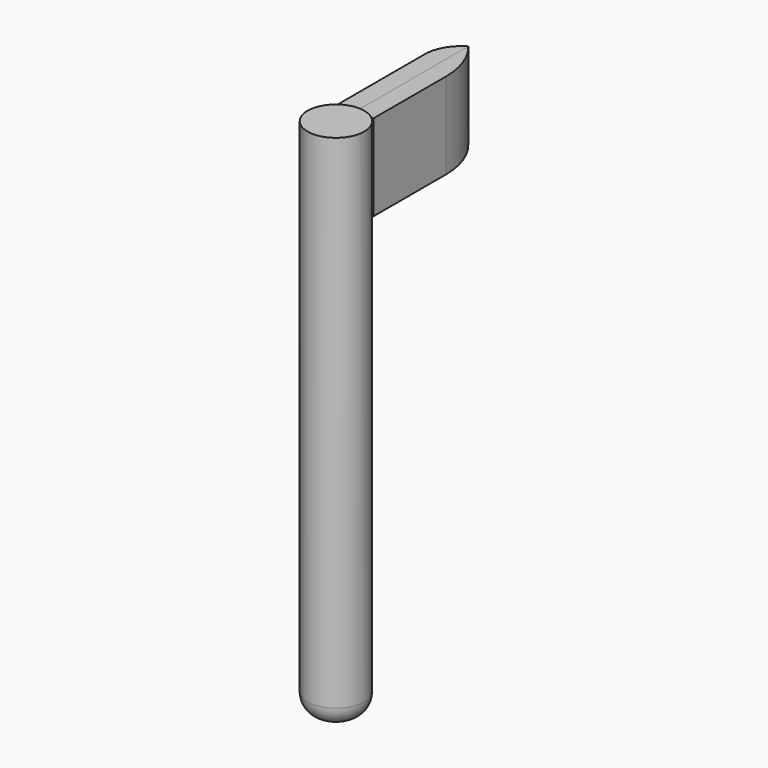
from build123d import *

# Parameters (mm, degrees)
F0_W        = 3.9413794875
F0_H        = 72.7184470743
F2_W        = 19.7068979032
F2_H        = 12.0212044567
F3_DEPTH    = 2.54
F4_T1_DEPTH = 47.2420593542
F5_DEPTH    = 2.54
F6_T1_DEPTH = 34.0182497128
F7_R        = 2.7594461018


# Not quite as in the source:
# - a fillet or chamfer that OpenCascade refuses, or shapes differently, is made with other operations: its cross-section is extruded or revolved along the edge and cut away or added


with BuildPart() as f1:
    # F0 (on Right) → F1 (revolve)
    with BuildSketch(Plane.YZ):
        with Locations((-32.3193110526, 6.9959471002)):
            Rectangle(F0_W, F0_H)
    revolve(axis=Axis((0, -30.3486213088, 6.9959471002), (0, 0, 1)))

    # F7
    f7_edges = [f1.edges().sort_by_distance(p)[0] for p in [
        (0, -26.407242, -29.363276),
    ]]
    fillet(f7_edges, radius=F7_R)


with BuildPart() as f3:
    # F2 (on Right) → F3 (new body)
    with BuildSketch(Plane.YZ):
        with Locations((-17.1450001653, 37.1475005522)):
            Rectangle(F2_W, F2_H)
    extrude(amount=F3_DEPTH)

    # F4: fillet of radius 11.0377844072 on 1 edges, made by hand

    # F4_s2 → F4_t1 (cut)
    with BuildSketch(Plane.XY.offset(13.5264708751)):
        with BuildLine():
            ThreePointArc((0, -7.2915512137), (1.8856012845, -10.5916620712), (2.54, -14.3357221932))
            Line((2.54, -14.3357221932), (2.54, -7.2915512137))
            Line((2.54, -7.2915512137), (0, -7.2915512137))
        make_face()
    extrude(amount=F4_T1_DEPTH, mode=Mode.SUBTRACT)


with BuildPart() as f5:
    # F2 (on Right) → F5 (new body)
    with BuildSketch(Plane.YZ):
        with Locations((-17.1450001653, 37.1475005522)):
            Rectangle(F2_W, F2_H)
    extrude(amount=-F5_DEPTH)

    # F6: fillet of radius 5.08 on 1 edges, made by hand

    # F6_s2 → F6_t1 (cut)
    with BuildSketch(Plane.XY.offset(20.1383756958)):
        with BuildLine():
            ThreePointArc((0, -7.2915512137), (-1.8594090512, -9.1509602649), (-2.54, -11.6909602649))
            Line((-2.54, -11.6909602649), (-2.54, -7.2915512137))
            Line((-2.54, -7.2915512137), (0, -7.2915512137))
        make_face()
    extrude(amount=F6_T1_DEPTH, mode=Mode.SUBTRACT)


solid = Compound([f1.part, f3.part, f5.part])
